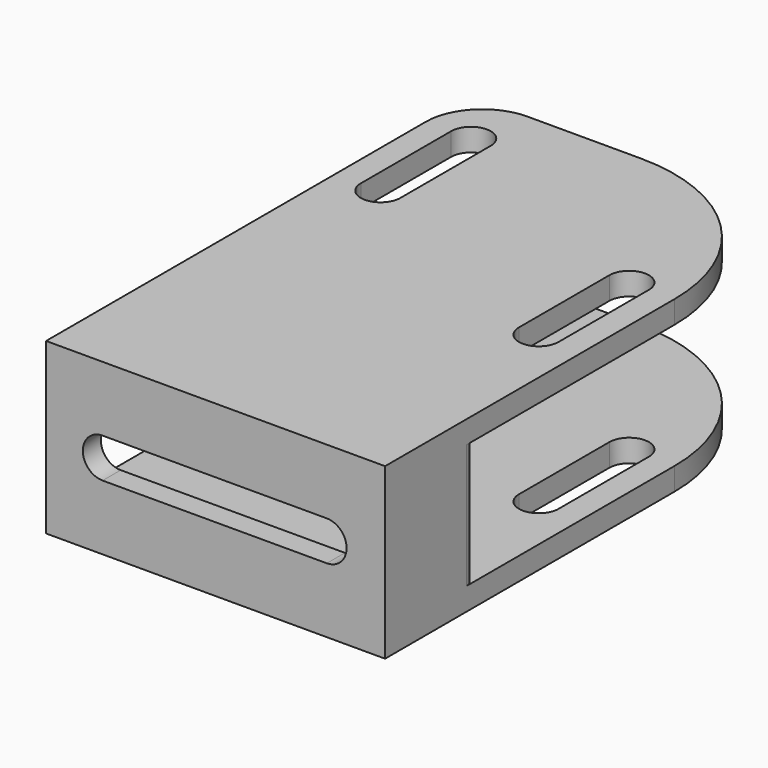
from build123d import *

# Parameters (mm, degrees)
F0_W     = 30
F0_H     = 45
F1_DEPTH = 2
F2_W     = 30
F2_H     = 2
F2_H_2   = 5.5
F3_DEPTH = 2
F6_DEPTH = 25
F7_W     = 8
F7_H     = 11
F8_DEPTH = 2
F9_R     = 15
F10_R    = 5
F11_R    = 0.99999


# Not quite as in the source:
# - a fillet or chamfer is up to 0.001 mm smaller than in the source, because OpenCascade refuses the exact size
# - ends of sketch curves that miss each other by under 0.0002 mm in the source are joined


with BuildPart() as f1:
    # F0 (on Top) → F1 (new body)
    with BuildSketch(Plane.XY):
        with Locations((-15, -22.5)):
            Rectangle(F0_W, F0_H)
        with BuildLine():
            ThreePointArc((-27.75, -5), (-26, -3.25), (-24.25, -5))
            Line((-24.25, -5), (-24.25, -15))
            ThreePointArc((-24.25, -15), (-26, -16.75), (-27.75, -15))
            Line((-27.75, -15), (-27.75, -5))
        make_face(mode=Mode.SUBTRACT)
        with BuildLine():
            Line((-2.25, -15), (-2.25, -25))
            ThreePointArc((-2.25, -25), (-4, -26.75), (-5.75, -25))
            Line((-5.75, -25), (-5.75, -15))
            ThreePointArc((-5.75, -15), (-4, -13.25), (-2.25, -15))
        make_face(mode=Mode.SUBTRACT)
    extrude(amount=F1_DEPTH)

    # F2 (on face) → F3 (join)
    with BuildSketch(Plane.XZ.offset(45)):
        with Locations((-15, 1)):
            Rectangle(F2_W, F2_H)
        with Locations((-15, 4.75)):
            Rectangle(F2_W, F2_H_2)
    extrude(amount=F3_DEPTH)

    # F4: F1 across face


with BuildPart() as f1_1:
    add(f1.part)
    add(f1.part.mirror(Plane(origin=(-15, -46, 7.5), x_dir=(1, 0, 0), z_dir=(0, 0, 1))))

    # F5 (on face) → F6 (cut)
    with BuildSketch(Plane(origin=(0, -45, 0), x_dir=(-1, 0, 0), z_dir=(0, 1, 0))):
        with BuildLine():
            ThreePointArc((5.1587387914, 9.2572143), (3.4087387914, 7.5072143), (5.1587387913, 5.7572143))
            Line((5.1587387913, 5.7572143), (25.0000000102, 5.7500001157))
            ThreePointArc((25.0000000102, 5.7500001157), (26.7500000102, 7.5), (25.0000000102, 9.25))
            Line((25.0000000102, 9.25), (5.1587387914, 9.2572143))
        make_face()
    extrude(amount=-F6_DEPTH, mode=Mode.SUBTRACT)

    # F7 (on face) → F8 (join)
    with BuildSketch(Plane.YZ):
        Polygon((-37, 13), (-37, 15), (-47, 15), (-47, 0), (-37, 0), (-37, 2), (-45, 2), (-45, 13), align=None)
        with Locations((-41, 7.5)):
            Rectangle(F7_W, F7_H)
    extrude(amount=-F8_DEPTH)

    # F9
    f9_edges = [f1_1.edges().sort_by_distance(p)[0] for p in [
        (0, 0, 1),
        (0, 0, 14),
    ]]
    fillet(f9_edges, radius=F9_R)

    # F10
    f10_edges = [f1_1.edges().sort_by_distance(p)[0] for p in [
        (-30, 0, 14),
        (-30, 0, 1),
    ]]
    fillet(f10_edges, radius=F10_R)

    # F11 (radius 1 in the source; OpenCascade refuses exactly that, so slightly less here)
    f11_edges = [f1_1.edges().sort_by_distance(p)[0] for p in [
        (-2, -37, 7.5),
        (0, -37, 7.5),
    ]]
    fillet(f11_edges, radius=F11_R)


solid = f1_1.part
